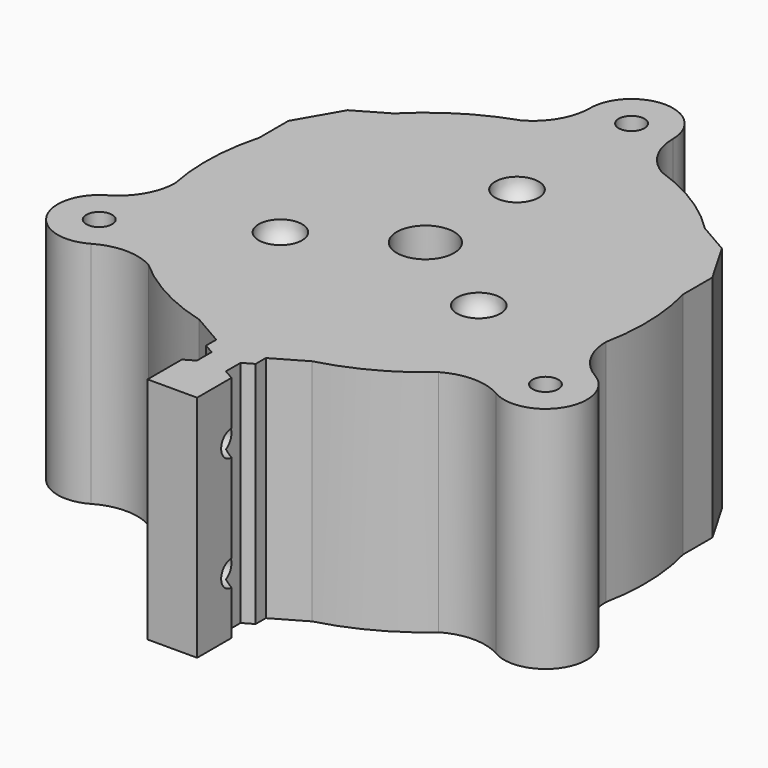
from build123d import *

# Parameters (mm, degrees)
F0_R             = 2.25
F0_R_2           = 33.35
F1_DEPTH         = 40
F2_R             = 33.35
F3_DEPTH         = 40
F5_DEPTH         = 5
F6_R             = 5
F7_DEPTH         = 6
F11_COPIES_COUNT = 3
F12_SIZE         = 5
F14_DEPTH        = 40
F15_R            = 2.25
F16_DEPTH        = 50.5522701892


# Not quite as in the source:
# - a pattern or mirror of a feature is missing from the dataset's text; its kind, count and spacing are read off the source's solid


with BuildPart() as f1:
    # F0 (on Top) → F1 (new body)
    with BuildSketch(Plane.XY):
        with BuildLine():
            ThreePointArc((-35.3461431703, -28.7786841774), (-30.3488782685, -27.4389385893), (-25.3508812473, -28.775950375))
            ThreePointArc((-25.3508812473, -28.775950375), (0, -38.35), (25.3508812473, -28.775950375))
            ThreePointArc((25.3508812473, -28.775950375), (30.3488782685, -27.4389385893), (35.3461431703, -28.7786841774))
            ThreePointArc((35.3461431703, -28.7786841774), (45.2498273477, -26.125), (42.5961431703, -16.2213158226))
            ThreePointArc((42.5961431703, -16.2213158226), (38.9372570055, -12.5634302623), (37.5961446665, -7.566531981))
            ThreePointArc((37.5961446665, -7.566531981), (33.2120742351, 19.175), (12.2452634191, 36.342482356))
            ThreePointArc((12.2452634191, 36.342482356), (8.588378737, 40.0023688516), (7.25, 45))
            ThreePointArc((7.25, 45), (0, 52.25), (-7.25, 45))
            ThreePointArc((-7.25, 45), (-8.588378737, 40.0023688516), (-12.2452634191, 36.342482356))
            ThreePointArc((-12.2452634191, 36.342482356), (-33.2120742351, 19.175), (-37.5961446665, -7.566531981))
            ThreePointArc((-37.5961446665, -7.566531981), (-38.9372570055, -12.5634302623), (-42.5961431703, -16.2213158226))
            ThreePointArc((-42.5961431703, -16.2213158226), (-45.2498273477, -26.125), (-35.3461431703, -28.7786841774))
        make_face()
        with Locations((-38.9711431703, -22.5)):
            Circle(F0_R, mode=Mode.SUBTRACT)
        with Locations((38.9711431703, -22.5)):
            Circle(F0_R, mode=Mode.SUBTRACT)
        Circle(F0_R_2, mode=Mode.SUBTRACT)
        with Locations((0, 45)):
            Circle(F0_R, mode=Mode.SUBTRACT)
    extrude(amount=F1_DEPTH)

    # F2 (on Top) → F3 (join)
    with BuildSketch(Plane.XY):
        Polygon((37.0225860118, -21.375), (37.0225860118, 21.375), (0, 42.75), (-37.0225860118, 21.375), (-37.0225860118, -21.375), (0, -42.75), align=None)
        Circle(F2_R, mode=Mode.SUBTRACT)
    extrude(amount=F3_DEPTH)

    # F4 (on Top) → F5 (cut)
    with BuildSketch(Plane.XY):
        with BuildLine():
            Line((-31.3188603972, -20.3913535578), (-30.4323380454, -19.8795196393))
            ThreePointArc((-30.4323380454, -19.8795196393), (0, -36.35), (30.4323380454, -19.8795196393))
            Line((30.4323380454, -19.8795196393), (31.3188603972, -20.3913535578))
            ThreePointArc((31.3188603972, -20.3913535578), (34.0509112048, -19.6593027502), (33.3188603972, -16.9272519427))
            Line((33.3188603972, -16.9272519427), (32.4323380454, -16.4154180242))
            ThreePointArc((32.4323380454, -16.4154180242), (31.4800234276, 18.175), (2, 36.2949376635))
            Line((2, 36.2949376635), (2, 37.3186055005))
            ThreePointArc((2, 37.3186055005), (0, 39.3186055005), (-2, 37.3186055005))
            Line((-2, 37.3186055005), (-2, 36.2949376635))
            ThreePointArc((-2, 36.2949376635), (-31.4800234276, 18.175), (-32.4323380454, -16.4154180242))
            Line((-32.4323380454, -16.4154180242), (-33.3188603972, -16.9272519427))
            ThreePointArc((-33.3188603972, -16.9272519427), (-34.0509112048, -19.6593027502), (-31.3188603972, -20.3913535578))
        make_face()
    extrude(amount=F5_DEPTH, mode=Mode.SUBTRACT)

    # F6 (on face) → F7 (join)
    with BuildSketch(Plane.XY.offset(40)):
        Polygon((37.0225860118, -21.375), (37.0225860118, 21.375), (0, 42.75), (-37.0225860118, 21.375), (-37.0225860118, -21.375), (0, -42.75), align=None)
        Circle(F6_R, mode=Mode.SUBTRACT)
    extrude(amount=-F7_DEPTH)

    # F8 (on Front) → F9 (revolve)
    with BuildSketch(Plane.XZ):
        with BuildLine():
            ThreePointArc((5, 32.9730571831), (23.5820111526, 23.5820111526), (32.9730571831, 5))
            Line((32.9730571831, 5), (38.3295804164, 5))
            Line((38.3295804164, 5), (38.3295804164, 34))
            Line((38.3295804164, 34), (5, 34))
            Line((5, 34), (5, 32.9730571831))
        make_face()
    revolve(axis=Axis((0, 0, 20), (0, 0, -1)))

    # F10 (on face) → F11 (revolve, cut)
    with BuildSketch(Plane.XY.offset(40)):
        with BuildLine():
            ThreePointArc((0, 16.2), (3.8, 20), (0, 23.8))
            Line((0, 23.8), (0, 16.2))
        make_face()
    f11 = revolve(axis=Axis((0, 20, 40), (0, -1, 0)), mode=Mode.SUBTRACT)

    # F11_copies: F11 ×3 about axis
    f11_copies_axis = Axis((0, 0, 0), (0, 0, 1))
    for i in range(1, F11_COPIES_COUNT):
        add(f11.rotate(f11_copies_axis, i * 360 / F11_COPIES_COUNT), mode=Mode.SUBTRACT)

    # F12
    f12_edges = [f1.edges().sort_by_distance(p)[0] for p in [
        (-37.022586, 21.375, 20),
        (0, -42.75, 20),
        (37.022586, 21.375, 20),
    ]]
    chamfer(f12_edges, length=F12_SIZE)

    # F13 (on Top) → F14 (join)
    with BuildSketch(Plane.XY):
        Polygon((4.3301270189, -40.25), (0, -40.25), (-4.3301270189, -40.25), (-4.3301270189, -42.4715390309), (-2.5301270189, -43.5107695155), (-2.5301270189, -46.7107695155), (-4.3301270189, -47.75), (-4.3301270189, -55.25), (0, -55.25), (4.3301270189, -55.25), (4.3301270189, -47.75), (2.5301270189, -46.7107695155), (2.5301270189, -43.5107695155), (4.3301270189, -42.4715390309), align=None)
    extrude(amount=F14_DEPTH)

    # F15 (on face) → F16 (cut, through all)
    with BuildSketch(Plane.YZ.offset(4.3301270189)):
        with Locations((-47.75, 10)):
            Circle(F15_R)
        with Locations((-47.75, 30)):
            Circle(F15_R)
    extrude(amount=-F16_DEPTH, mode=Mode.SUBTRACT)


solid = f1.part
